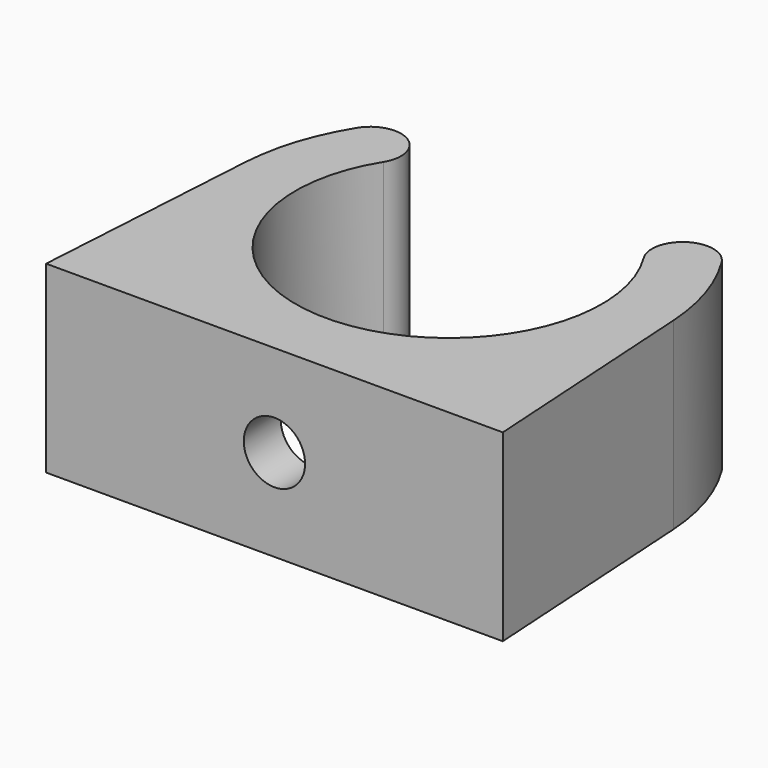
from build123d import *

# Parameters (mm, degrees)
F1_DEPTH       = 15
F4_D           = 5
F4_START       = 12.5000001
F4_CBORE_D     = 10
F4_CBORE_DEPTH = 1.5


# Not quite as in the source:
# - a feature of the source that left no trace in its solid (it failed there, or was rolled back) is left out


with BuildPart() as f1:
    # F0 (on Top) → F1 (new body)
    with BuildSketch(Plane.XY):
        with BuildLine():
            ThreePointArc((10.6047668571, 35.4310178135), (0.0084014235, 16.3137009448), (-10.6136524588, 35.4167566161))
            ThreePointArc((-10.6136524588, 35.4167566161), (-11.4157712516, 38.8600988068), (-14.8591134423, 38.057980014))
            ThreePointArc((-14.8591134423, 38.057980014), (-16.6714054435, 34.1348108377), (-17.4670460885, 29.8871509353))
            Line((-17.4670460885, 29.8871509353), (-18.6252595091, 11.0408943146))
            Line((-18.6252595091, 11.0408943146), (18.6252595091, 11.0408943146))
            Line((18.6252595091, 11.0408943146), (17.4670460885, 29.8871509353))
            ThreePointArc((17.4670460885, 29.8871509353), (16.6678252842, 34.1460147189), (14.8466735999, 38.0779456904))
            ThreePointArc((14.8466735999, 38.0779456904), (11.4022562901, 38.8754351234), (10.6047668571, 35.4310178135))
        make_face()
    extrude(amount=F1_DEPTH)

    # F4 (through all)
    # its depths count from where the whole tool has entered the part; down to there all is cleared
    with Locations(Plane(origin=(0, 28.8136981214, 0), x_dir=(-1, 0, 0), z_dir=(0, 1, 0)).offset(-F4_START)):
        with Locations((0, 7.5)):
            CounterBoreHole(F4_D / 2, F4_CBORE_D / 2, F4_CBORE_DEPTH)


solid = f1.part
